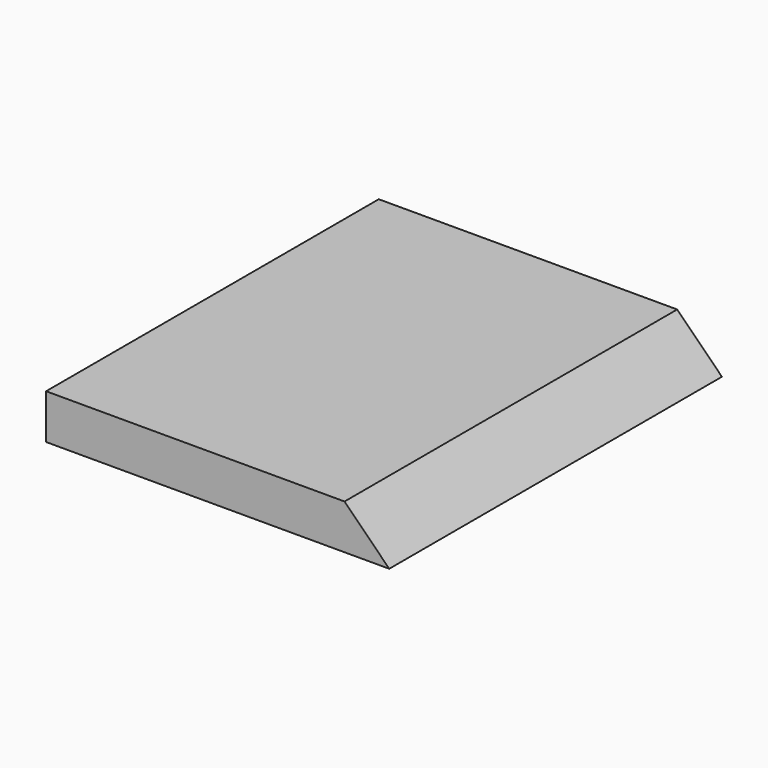
from build123d import *

# Parameters (mm, degrees)
F0_W     = 76.7452418804
F0_H     = 92.9985865951
F1_DEPTH = 5
F3_SIZE  = 9.99999


# Not quite as in the source:
# - a fillet or chamfer is up to 0.001 mm smaller than in the source, because OpenCascade refuses the exact size


with BuildPart() as f1:
    # F0 (on Top) → F1 (new body, symmetric)
    with BuildSketch(Plane.XY):
        with Locations((38.3726209402, 46.4992932975)):
            Rectangle(F0_W, F0_H)
    extrude(amount=F1_DEPTH, both=True)

    # F3 (size 10 in the source; OpenCascade refuses exactly that, so slightly less here)
    f3_edges = [f1.edges().sort_by_distance(p)[0] for p in [
        (76.745242, 46.499293, 5),
    ]]
    chamfer(f3_edges, length=F3_SIZE)


solid = f1.part
